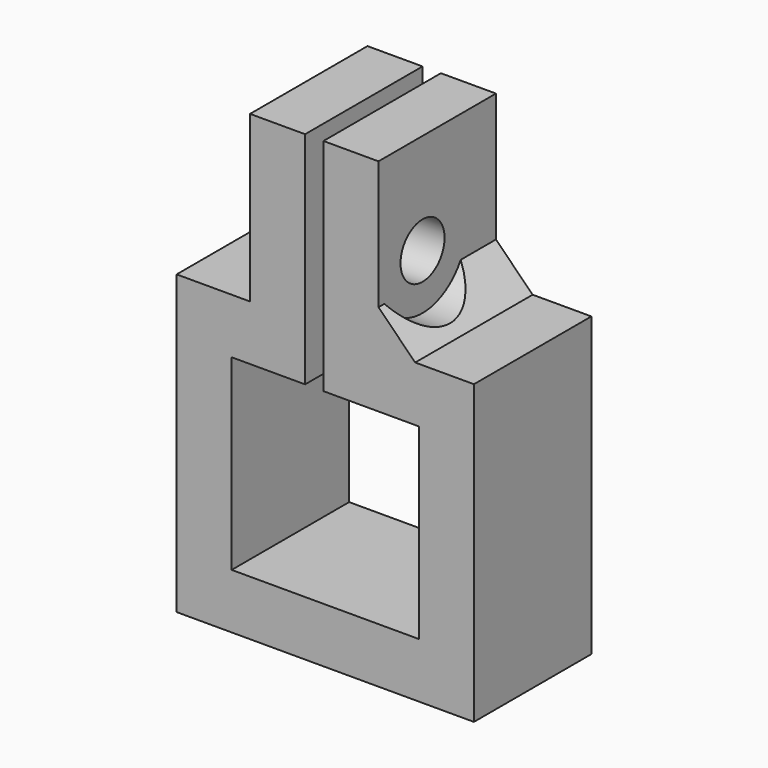
from build123d import *

# Parameters (mm, degrees)
F1_DEPTH = 8
F2_R     = 1.5
F3_DEPTH = 12.5
F4_SIZE  = 1.99999
F5_R     = 3
F6_DEPTH = 4
F8_DEPTH = 2


# Not quite as in the source:
# - a fillet or chamfer is up to 0.001 mm smaller than in the source, because OpenCascade refuses the exact size


with BuildPart() as f1:
    # F0 (on Front) → F1 (new body)
    with BuildSketch(Plane.XZ):
        Polygon((5.1, 5.1), (5.1, -5.1), (-5.1, -5.1), (-5.1, 5.1), (-4.1, 5.1), (-1.1, 5.1), (-1.1, 8.1), (-1.1, 17.1), (-4.1, 17.1), (-4.1, 8.1), (-5.1, 8.1), (-8.1, 8.1), (-8.1, -8.1), (8.1, -8.1), (8.1, 8.1), (2.9, 8.1), (2.9, 17.1), (-0.1, 17.1), (-0.1, 8.1), (-0.1, 5.1), align=None)
    extrude(amount=F1_DEPTH)

    # F2 (on face) → F3 (cut, symmetric)
    with BuildSketch(Plane.YZ.offset(-1.1)):
        with Locations((-5, 11.6)):
            Circle(F2_R)
    extrude(amount=F3_DEPTH, both=True, mode=Mode.SUBTRACT)

    # F4 (size 2 in the source; OpenCascade refuses exactly that, so slightly less here)
    f4_edges = [f1.edges().sort_by_distance(p)[0] for p in [
        (2.9, -4, 8.1),
    ]]
    chamfer(f4_edges, length=F4_SIZE)

    # F5 (on face) → F6 (cut)
    with BuildSketch(Plane.YZ.offset(2.9)):
        with Locations((-5, 11.6)):
            Circle(F5_R)
    extrude(amount=F6_DEPTH, mode=Mode.SUBTRACT)

    # F7 (on face) → F8 (join)
    with BuildSketch(Plane(origin=(0, 0, 0), x_dir=(-1, 0, 0), z_dir=(0, 1, 0))):
        Polygon((4.1, 8.1), (8.1, 8.1), (4.1, 12.6), align=None)
    extrude(amount=-F8_DEPTH)


solid = f1.part
